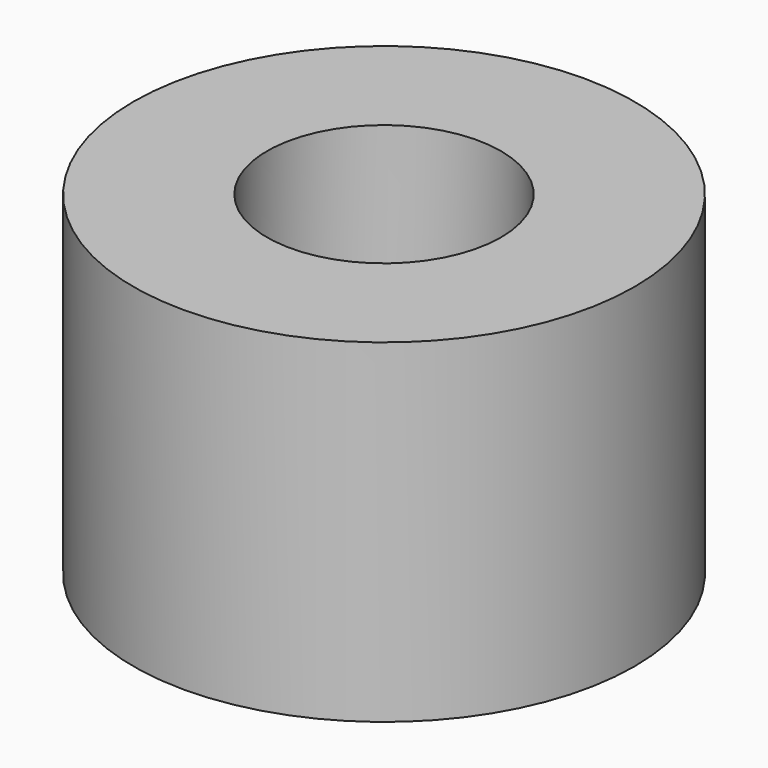
from build123d import *

# Parameters (mm, degrees)
F0_R     = 3.75
F0_R_2   = 1.75
F1_DEPTH = 3.8
F3_DEPTH = 2.5
F4_DEPTH = 1.2


with BuildPart() as f1:
    # F0 (on Top) → F1 (new body)
    with BuildSketch(Plane.XY):
        with Locations((56.9799989462, -33.0372825265)):
            Circle(F0_R)
        with Locations((56.9799989462, -33.0372825265)):
            Circle(F0_R_2, mode=Mode.SUBTRACT)
    extrude(amount=F1_DEPTH)

    # F2 (on face) → F3 (cut)
    with BuildSketch(Plane(origin=(0, 0, 0), x_dir=(1, 0, 0), z_dir=(0, 0, -1))):
        Polygon((59.8799989462, 31.3629667458), (59.8799989462, 34.7115983071), (56.9799989462, 36.3859140878), (54.0799989462, 34.7115983071), (54.0799989462, 31.3629667458), (56.9799989462, 29.6886509652), align=None)
    extrude(amount=-F3_DEPTH, mode=Mode.SUBTRACT)

    # F4 (add): a face of the model
    f4_faces = [f1.faces().sort_by_distance(p)[0] for p in [
        (53.3360649634, -33.0372825265, 3.8),
    ]]
    extrude(f4_faces, amount=F4_DEPTH)


solid = f1.part
